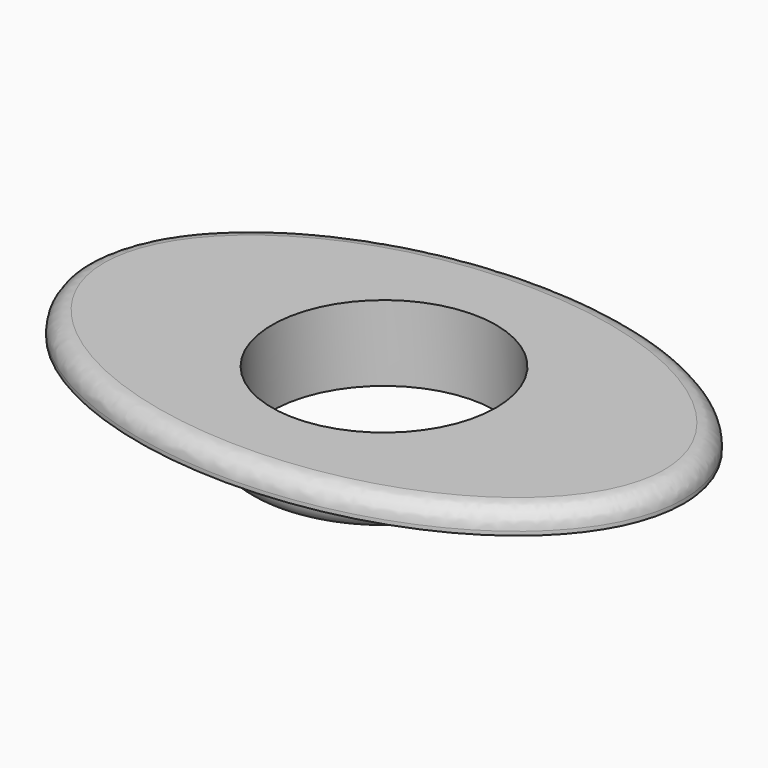
from build123d import *

# Parameters (mm, degrees)
F0_R     = 4.3
F1_DEPTH = 2.9
F2_R     = 5.3
F3_DEPTH = 2
F4_R     = 0.75


# Not quite as in the source:
# - a feature names something its author has since deleted; it is built from what else it names


with BuildPart() as f1:
    # F0 (on Top) → F1 (new body)
    with BuildSketch(Plane.XY):
        with BuildLine():
            add(Edge.make_bspline(
                [(11.5, 0), (11.5, 12.9903810568), (-5.75, 6.4951905284), (-23, 0), (-5.75, -6.4951905284), (11.5, -12.9903810568), (11.5, 0)],
                knots=[0, 0, 0, 2.0943951024, 2.0943951024, 4.1887902048, 4.1887902048, 6.2831853072, 6.2831853072, 6.2831853072], degree=2, weights=[1, 0.5, 1, 0.5, 1, 0.5, 1]))
        make_face()
        Circle(F0_R, mode=Mode.SUBTRACT)
    extrude(amount=-F1_DEPTH)

    # F2 (on face) → F3 (cut)
    with BuildSketch(Plane(origin=(0, 0, -2.9), x_dir=(1, 0, 0), z_dir=(0, 0, -1))):
        with BuildLine():
            add(Edge.make_bspline(
                [(11.5, 0), (11.5, 12.9903810568), (-5.75, 6.4951905284), (-23, 0), (-5.75, -6.4951905284), (11.5, -12.9903810568), (11.5, 0)],
                knots=[0, 0, 0, 2.0943951024, 2.0943951024, 4.1887902048, 4.1887902048, 6.2831853072, 6.2831853072, 6.2831853072], degree=2, weights=[1, 0.5, 1, 0.5, 1, 0.5, 1]))
        make_face()
        Circle(F2_R, mode=Mode.SUBTRACT)
    extrude(amount=-F3_DEPTH, mode=Mode.SUBTRACT)

    # F4
    f4_edges = [f1.edges().sort_by_distance(p)[0] for p in [
        (-11.5, 0, 0),
        (-5.3, 0, -2.9),
    ]]
    fillet(f4_edges, radius=F4_R)


solid = f1.part
